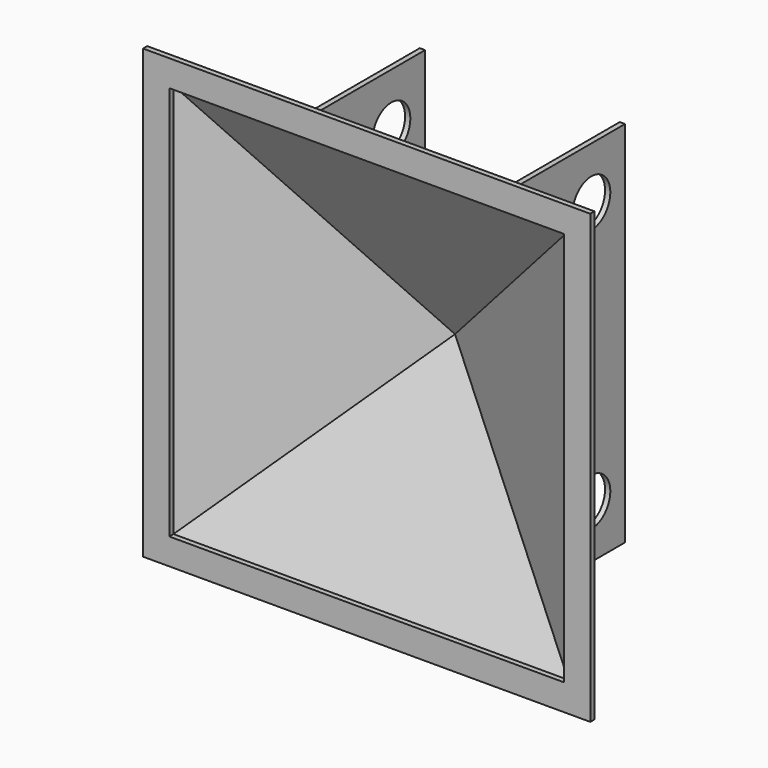
from build123d import *

# Parameters (mm, degrees)
F0_W      = 75
F0_H      = 75
F4_T      = 1
F0_W_2    = 85
F0_H_2    = 85
F5_DEPTH  = 1
F7_W      = 1
F7_H      = 70
F9_R      = 4.5
F10_DEPTH = 62.001


# Not quite as in the source:
# - a pattern or mirror of a feature is missing from the dataset's text; its kind, count and spacing are read off the source's solid


with BuildPart() as f3:
    # F0 (on Front) → F3 section 0
    with BuildSketch(Plane.XZ, mode=Mode.PRIVATE) as f3_s0:
        Rectangle(F0_W, F0_H)
    loft([f3_s0.sketch, Vertex(0, 20, 0)])

    # F4
    f4_openings = [f3.faces().sort_by_distance(p)[0] for p in [
        (0, 0, 0),
    ]]
    offset(amount=F4_T, openings=f4_openings, kind=Kind.INTERSECTION)

    # F0 (on Front) → F5 (join)
    with BuildSketch(Plane.XZ):
        Rectangle(F0_W_2, F0_H_2)
        Rectangle(F0_W, F0_H, mode=Mode.SUBTRACT)
    extrude(amount=F5_DEPTH)

    # F7 (on offset) → F8 (join, up to the next surface of F3)
    with BuildSketch(Plane.XZ.offset(-36)):
        with Locations((-19, 0)):
            Rectangle(F7_W, F7_H)
    f8 = extrude(until=Until.NEXT)

    # F8_copies: F8 across plane
    add(f8.mirror(Plane(origin=(0, 0, 0), x_dir=(0, 0, 1), z_dir=(1, 0, 0))))

    # F9 (on face) → F10 (cut, through all)
    with BuildSketch(Plane(origin=(-19.5, 0, 0), x_dir=(0, -1, 0), z_dir=(-1, 0, 0))):
        with Locations((-28, -25)):
            Circle(F9_R)
        with Locations((-28, 25)):
            Circle(F9_R)
    extrude(amount=-F10_DEPTH, mode=Mode.SUBTRACT)


solid = f3.part
